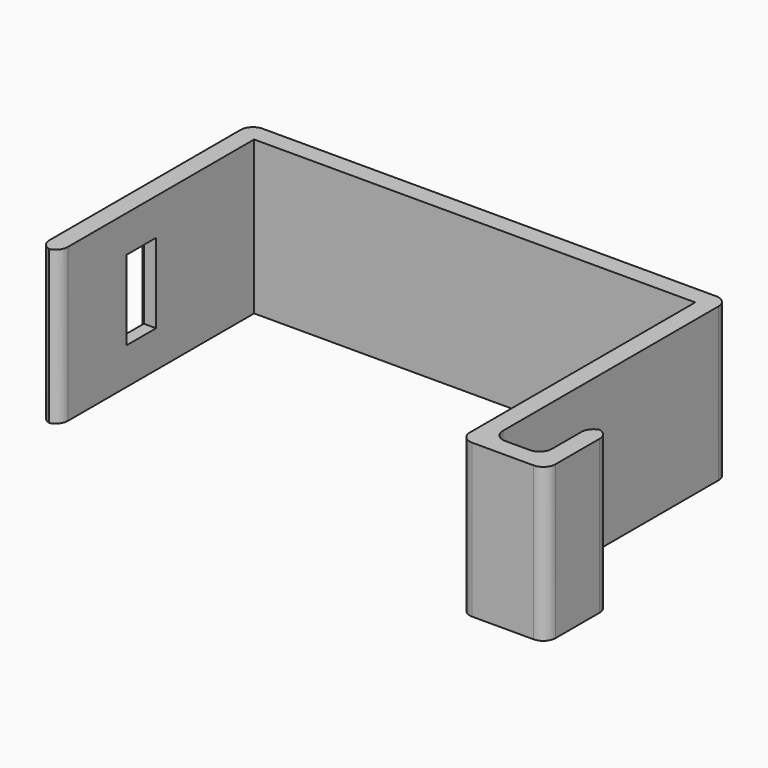
from build123d import *

# Parameters (mm, degrees)
F1_DEPTH    = 25
F2_W        = 6
F2_H        = 13
F3_DEPTH    = 12.5
F4_SIZE2    = 1
F4_SIZE     = 1
F5_T1_DEPTH = 25
F5_T3_DEPTH = 35


# Not quite as in the source:
# - a fillet or chamfer that OpenCascade refuses, or shapes differently, is made with other operations: its cross-section is extruded or revolved along the edge and cut away or added


with BuildPart() as f1:
    # F0 (on Top) → F1 (new body)
    with BuildSketch(Plane.XY):
        Polygon((-55.1361331344, -5), (-52.1361331344, -5), (-52.1361331344, 35), (19.8638668656, 35), (19.8638668656, -10), (19.8638668656, -13), (30.8638668656, -13), (33.8638668656, -13), (33.8638668656, -10), (33.8638668656, 0), (30.8638668656, 0), (30.8638668656, -10), (22.8638668656, -10), (22.8638668656, 38), (-55.1361331344, 38), align=None)
    extrude(amount=F1_DEPTH)

    # F2 (on face) → F3 (cut, symmetric)
    with BuildSketch(Plane(origin=(-55.1361331344, 0, 0), x_dir=(0, -1, 0), z_dir=(-1, 0, 0))):
        with Locations((-12, 12.5)):
            Rectangle(F2_W, F2_H)
    extrude(amount=F3_DEPTH, both=True, mode=Mode.SUBTRACT)

    # F4
    f4_edges = [f1.edges().sort_by_distance(p)[0] for p in [
        (-55.136133, 12, 19),
        (-55.136133, 15, 12.5),
        (-55.136133, 9, 12.5),
        (-55.136133, 12, 6),
    ]]
    chamfer(f4_edges, length=F4_SIZE, length2=F4_SIZE2)

    # F5: fillet of radius 2 on 10 edges, made by hand

    # F5_s2 → F5_t1 (join)
    with BuildSketch(Plane.XY):
        with BuildLine():
            ThreePointArc((22.8638668656, -8), (23.4496533033, -9.4142135624), (24.8638668656, -10))
            Line((24.8638668656, -10), (22.8638668656, -10))
            Line((22.8638668656, -10), (22.8638668656, -8))
        make_face()
        with BuildLine():
            ThreePointArc((30.8638668656, -8), (30.278080428, -9.4142135624), (28.8638668656, -10))
            Line((28.8638668656, -10), (30.8638668656, -10))
            Line((30.8638668656, -10), (30.8638668656, -8))
        make_face()
    extrude(amount=F5_T1_DEPTH)

    # F5_s4 → F5_t3 (cut)
    with BuildSketch(Plane.XY.offset(-5)):
        with BuildLine():
            ThreePointArc((-55.1361331344, 36), (-54.5503466967, 37.4142135624), (-53.1361331344, 38))
            Line((-53.1361331344, 38), (-55.1361331344, 38))
            Line((-55.1361331344, 38), (-55.1361331344, 36))
        make_face()
        with BuildLine():
            ThreePointArc((20.8638668656, 38), (22.278080428, 37.4142135624), (22.8638668656, 36))
            Line((22.8638668656, 36), (22.8638668656, 38))
            Line((22.8638668656, 38), (20.8638668656, 38))
        make_face()
        with BuildLine():
            ThreePointArc((19.8638668656, -11), (20.4496533033, -12.4142135624), (21.8638668656, -13))
            Line((21.8638668656, -13), (19.8638668656, -13))
            Line((19.8638668656, -13), (19.8638668656, -11))
        make_face()
        with BuildLine():
            ThreePointArc((31.8638668656, -13), (33.278080428, -12.4142135624), (33.8638668656, -11))
            Line((33.8638668656, -11), (33.8638668656, -13))
            Line((33.8638668656, -13), (31.8638668656, -13))
        make_face()
        with BuildLine():
            ThreePointArc((33.8638668656, -2), (33.278080428, -0.5857864376), (31.8638668656, 0))
            Line((31.8638668656, 0), (33.8638668656, 0))
            Line((33.8638668656, 0), (33.8638668656, -2))
        make_face()
        with BuildLine():
            ThreePointArc((32.8638668656, 0), (31.4496533033, -0.5857864376), (30.8638668656, -2))
            Line((30.8638668656, -2), (30.8638668656, 0))
            Line((30.8638668656, 0), (32.8638668656, 0))
        make_face()
        with BuildLine():
            ThreePointArc((-55.1361331344, -3), (-54.5503466967, -4.4142135624), (-53.1361331344, -5))
            Line((-53.1361331344, -5), (-55.1361331344, -5))
            Line((-55.1361331344, -5), (-55.1361331344, -3))
        make_face()
        with BuildLine():
            ThreePointArc((-54.1361331344, -5), (-52.721919572, -4.4142135624), (-52.1361331344, -3))
            Line((-52.1361331344, -3), (-52.1361331344, -5))
            Line((-52.1361331344, -5), (-54.1361331344, -5))
        make_face()
    extrude(amount=F5_T3_DEPTH, mode=Mode.SUBTRACT)


solid = f1.part
